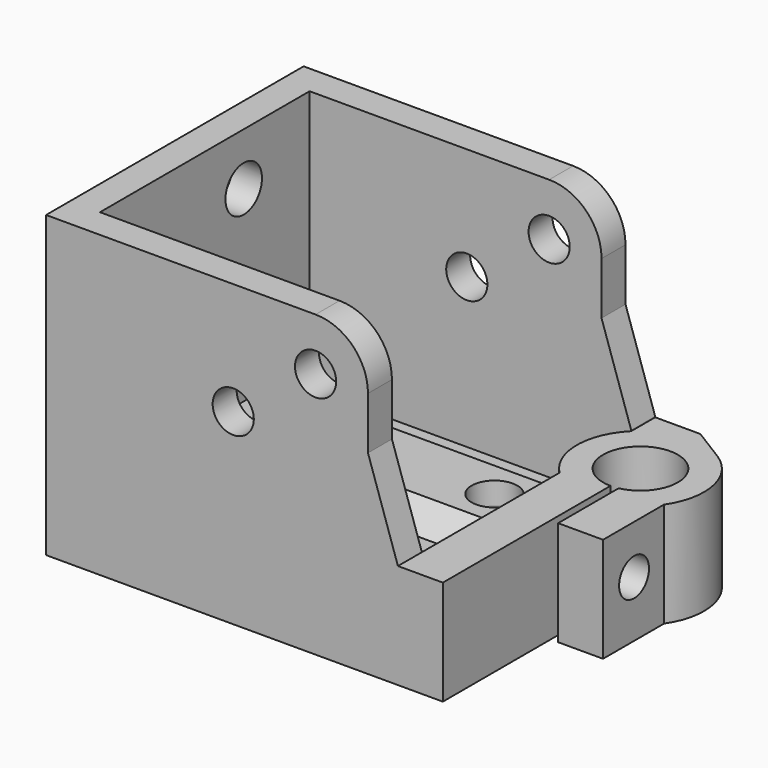
from build123d import *

# Parameters (mm, degrees)
F0_W           = 53
F0_H           = 43
F1_DEPTH       = 5
F3_DEPTH       = 9
F3_DEPTH_BACK  = 5
F4_DEPTH       = 25
F6_DEPTH       = 35
F7_R           = 2.75
F8_DEPTH       = 43.001
F10_DEPTH      = 3
F10_DEPTH_BACK = 6
F11_R          = 2.5
F12_DEPTH      = 25
F13_W          = 37.7532099868
F13_H          = 10
F14_DEPTH      = 3
F15_R          = 3.05
F16_DEPTH      = 25
F16_DEPTH_BACK = 25
F17_SIZE       = 2.99999
F18_R          = 3.05
F19_DEPTH      = 25


# Not quite as in the source:
# - a fillet or chamfer is up to 0.001 mm smaller than in the source, because OpenCascade refuses the exact size


with BuildPart() as f1:
    # F0 (on Top) → F1 (new body)
    with BuildSketch(Plane.XY):
        with Locations((26.5, 21.5)):
            Rectangle(F0_W, F0_H)
    extrude(amount=F1_DEPTH)

    # F2 (on face) → F3 (join, two sides)
    with BuildSketch(Plane.XY.offset(5)) as f3_sk:
        with BuildLine():
            Line((47, 0), (53, 0))
            Line((53, 0), (53, 24.5))
            Line((53, 24.5), (53, 28))
            ThreePointArc((53, 28), (52.49745519, 37.974680765), (54, 28.1010205144))
            Line((54, 28.1010205144), (54, 24.5590284919))
            Line((54, 24.5590284919), (54, 18))
            Line((54, 18), (60, 18))
            Line((60, 18), (60, 25.8046761155))
            Line((60, 25.8046761155), (60, 28.1781746195))
            ThreePointArc((60, 28.1781746195), (61.3195930877, 34.7419445616), (57.477652845, 40.225))
            Line((57.477652845, 40.225), (53, 43))
            Line((53, 43), (47, 43))
            Line((47, 43), (46.9, 43))
            Line((46.9, 43), (46.9, 38.9194594348))
            ThreePointArc((46.9, 38.9194594348), (44.5002980841, 32.9288147474), (47, 26.9792027106))
            Line((47, 26.9792027106), (47, 0))
        make_face()
    extrude(amount=F3_DEPTH)
    extrude(f3_sk.sketch, amount=-F3_DEPTH_BACK)

    # F2 (on face) → F4 (cut)
    with BuildSketch(Plane.XY.offset(5)):
        with BuildLine():
            ThreePointArc((53, 38), (48, 33), (53, 28))
            Line((53, 28), (53, 28.1010205144))
            Line((53, 28.1010205144), (53, 38))
        make_face()
    extrude(amount=-F4_DEPTH, mode=Mode.SUBTRACT)

    # F5 (on face) → F6 (join)
    with BuildSketch(Plane.XY.offset(5)):
        Polygon((0, 43), (0, 0), (47, 0), (47, 4.00000019), (4.00000019, 4.00000019), (4.00000019, 38.99999981), (46.9636693597, 38.99999981), (46.9636693597, 43), align=None)
    extrude(amount=F6_DEPTH)

    # F7 (on face) → F8 (cut, through all)
    with BuildSketch(Plane.XZ):
        with Locations((36, 33)):
            Circle(F7_R)
        with Locations((25, 25)):
            Circle(F7_R)
        with BuildLine():
            ThreePointArc((36, 40), (40.9497474683, 37.9497474683), (43, 33))
            Line((43, 33), (43, 26))
            Line((43, 26), (47, 14))
            Line((47, 14), (47, 40))
            Line((47, 40), (36, 40))
        make_face()
    extrude(amount=-F8_DEPTH, mode=Mode.SUBTRACT)

    # F9 (on face) → F10 (cut, two sides)
    with BuildSketch(Plane(origin=(47, 0, 0), x_dir=(0, -1, 0), z_dir=(-1, 0, 0))) as f10_sk:
        Polygon((-18.9281746195, 5.0462613559), (-18.9281746195, 9.9537386441), (-23.1781746195, 12.4074772881), (-27.4281746195, 9.9537386441), (-27.4281746195, 5.0462613559), (-23.1781746195, 2.5925227119), align=None)
    extrude(amount=-F10_DEPTH, mode=Mode.SUBTRACT)
    extrude(f10_sk.sketch, amount=F10_DEPTH_BACK, mode=Mode.SUBTRACT)

    # F11 (on face) → F12 (cut)
    with BuildSketch(Plane.YZ.offset(60)):
        with Locations((23.1781746195, 7.5)):
            Circle(F11_R)
    extrude(amount=-F12_DEPTH, mode=Mode.SUBTRACT)

    # F13 (on face) → F14 (join)
    with BuildSketch(Plane.XY.offset(5)):
        with Locations((22.1233950066, 28)):
            Rectangle(F13_W, F13_H)
    extrude(amount=F14_DEPTH)

    # F15 (on face) → F16 (cut, two sides)
    with BuildSketch(Plane.XY.offset(5)) as f16_sk:
        with Locations((15.5, 28)):
            Circle(F15_R)
        with Locations((37.5, 28)):
            Circle(F15_R)
    extrude(amount=-F16_DEPTH, mode=Mode.SUBTRACT)
    extrude(f16_sk.sketch, amount=F16_DEPTH_BACK, mode=Mode.SUBTRACT)

    # F17 (size 3 in the source; OpenCascade refuses exactly that, so slightly less here)
    f17_edges = [f1.edges().sort_by_distance(p)[0] for p in [
        (22.5, 23, 5),
        (22.5, 33, 5),
    ]]
    chamfer(f17_edges, length=F17_SIZE)

    # F18 (on face) → F19 (cut)
    with BuildSketch(Plane(origin=(0, 0, 0), x_dir=(0, -1, 0), z_dir=(-1, 0, 0))):
        with Locations((-28, 33)):
            Circle(F18_R)
    extrude(amount=-F19_DEPTH, mode=Mode.SUBTRACT)


solid = f1.part
